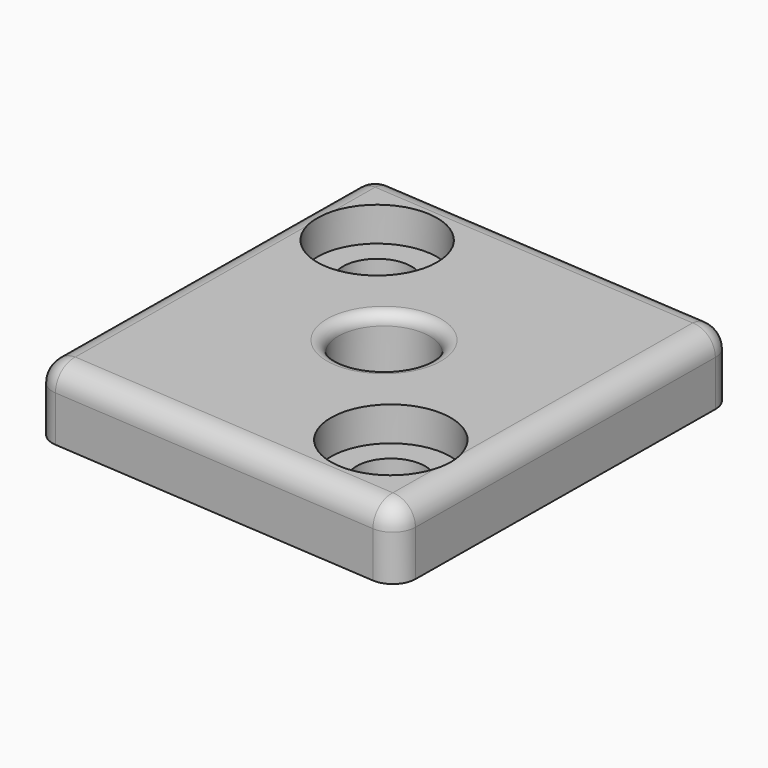
from build123d import *

# Parameters (mm, degrees)
F0_R         = 2.625
F0_R_2       = 2
F0_R_3       = 1.5
F1_DEPTH     = 3
F2_R         = 2.625
F2_R_2       = 1.5
F3_DEPTH     = 1.5
F4_T1_DEPTH  = 16.2344954865
F4_T3_DEPTH  = 14.8006020278
F4_T5_DEPTH  = 16.2344954865
F4_T7_DEPTH  = 14.8006020278
F4_T9_DEPTH  = 4.3472443006
F4_T11_DEPTH = 4.6626968477
F4_T16_DEPTH = 1
F4_T22_DEPTH = 1
F4_T28_DEPTH = 1
F4_T34_DEPTH = 1
F5_R         = 0.5


# Not quite as in the source:
# - a fillet or chamfer that OpenCascade refuses, or shapes differently, is made with other operations: its cross-section is extruded or revolved along the edge and cut away or added


with BuildPart() as f1:
    # F0 (on Top) → F1 (new body)
    with BuildSketch(Plane.XY):
        Polygon((8.4645454874, 8.5124193832), (-8.2962074114, 9.7252756798), (-8.4645454874, -8.5124193832), (8.2962074114, -9.7252756798), align=None)
        with Locations((4.8033426305, -5.6307453454)):
            Circle(F0_R, mode=Mode.SUBTRACT)
        Polygon((-2.3040371523, -3.3198032774), (-4.02705255, 0.3354530665), (-1.7230153977, 3.6552563439), (2.3040371523, 3.3198032774), (4.02705255, -0.3354530665), (1.7230153977, -3.6552563439), align=None, mode=Mode.SUBTRACT)
        with Locations((-4.8033426305, 5.6307453454)):
            Circle(F0_R, mode=Mode.SUBTRACT)
        Polygon((-1.7230153977, 3.6552563439), (-4.02705255, 0.3354530665), (-2.3040371523, -3.3198032774), (1.7230153977, -3.6552563439), (4.02705255, -0.3354530665), (2.3040371523, 3.3198032774), align=None)
        Circle(F0_R_2, mode=Mode.SUBTRACT)
        with Locations((-4.8033426305, 5.6307453454)):
            Circle(F0_R)
        with Locations((-4.8033426305, 5.6307453454)):
            Circle(F0_R_3, mode=Mode.SUBTRACT)
        with Locations((4.8033426305, -5.6307453454)):
            Circle(F0_R)
        with Locations((4.8033426305, -5.6307453454)):
            Circle(F0_R_3, mode=Mode.SUBTRACT)
    extrude(amount=F1_DEPTH)

    # F2 (on face) → F3 (cut)
    with BuildSketch(Plane.XY.offset(3)):
        with Locations((-4.8033426305, 5.6307453454)):
            Circle(F2_R)
        with Locations((-4.8033426305, 5.6307453454)):
            Circle(F2_R_2, mode=Mode.SUBTRACT)
        with Locations((4.8033426305, -5.6307453454)):
            Circle(F2_R)
        with Locations((4.8033426305, -5.6307453454)):
            Circle(F2_R_2, mode=Mode.SUBTRACT)
    extrude(amount=-F3_DEPTH, mode=Mode.SUBTRACT)

    # F4: fillet of radius 1 on 8 edges, made by hand

    # F4_s2 → F4_t1 (cut)
    with BuildSketch(Plane(origin=(0.0792216076, 8.582844455, 0), x_dir=(0, 0, 1), z_dir=(-0.0092298344, -0.9999574042, 0))):
        with BuildLine():
            ThreePointArc((2, 8.3856167117), (2.7071067812, 8.0927234929), (3, 7.3856167117))
            Line((3, 7.3856167117), (3, 8.3856167117))
            Line((3, 8.3856167117), (2, 8.3856167117))
        make_face()
    extrude(amount=F4_T1_DEPTH, mode=Mode.SUBTRACT)

    # F4_s4 → F4_t3 (cut)
    with BuildSketch(Plane(origin=(6.8712291985, -0.4972219118, 0), x_dir=(0, 0, 1), z_dir=(-0.9973920448, 0.0721741576, 0))):
        with BuildLine():
            ThreePointArc((3, 8.1011408148), (2.7071067812, 8.808247596), (2, 9.1011408148))
            Line((2, 9.1011408148), (3, 9.1011408148))
            Line((3, 9.1011408148), (3, 8.1011408148))
        make_face()
    extrude(amount=F4_T3_DEPTH, mode=Mode.SUBTRACT)

    # F4_s6 → F4_t5 (cut)
    with BuildSketch(Plane(origin=(-0.0792216076, -8.582844455, 0), x_dir=(0, 0, 1), z_dir=(0.0092298344, 0.9999574042, 0))):
        with BuildLine():
            ThreePointArc((2, 8.3856167117), (2.7071067812, 8.0927234929), (3, 7.3856167117))
            Line((3, 7.3856167117), (3, 8.3856167117))
            Line((3, 8.3856167117), (2, 8.3856167117))
        make_face()
    extrude(amount=F4_T5_DEPTH, mode=Mode.SUBTRACT)

    # F4_s8 → F4_t7 (cut)
    with BuildSketch(Plane(origin=(-6.8712291985, 0.4972219118, 0), x_dir=(0, 0, 1), z_dir=(0.9973920448, -0.0721741576, 0))):
        with BuildLine():
            ThreePointArc((2, 9.1011408148), (2.7071067812, 8.808247596), (3, 8.1011408148))
            Line((3, 8.1011408148), (3, 9.1011408148))
            Line((3, 9.1011408148), (2, 9.1011408148))
        make_face()
    extrude(amount=F4_T7_DEPTH, mode=Mode.SUBTRACT)

    # F4_s10 → F4_t9 (cut)
    with BuildSketch(Plane.XY.offset(-2.3472443006)):
        with BuildLine():
            ThreePointArc((8.4558796169, 7.573561656), (8.1912373991, 8.2605167863), (7.5280963703, 8.5801835352))
            Line((7.5280963703, 8.5801835352), (8.4645454874, 8.5124193832))
            Line((8.4645454874, 8.5124193832), (8.4558796169, 7.573561656))
        make_face()
        with BuildLine():
            ThreePointArc((-7.5280963703, -8.5801835352), (-8.1912373991, -8.2605167863), (-8.4558796169, -7.573561656))
            Line((-8.4558796169, -7.573561656), (-8.4645454874, -8.5124193832))
            Line((-8.4645454874, -8.5124193832), (-7.5280963703, -8.5801835352))
        make_face()
    extrude(amount=F4_T9_DEPTH, mode=Mode.SUBTRACT)

    # F4_s12 → F4_t11 (cut)
    with BuildSketch(Plane.XY.offset(-2.6626968477)):
        with BuildLine():
            ThreePointArc((7.23390635, -9.648404519), (7.9838058035, -9.3863276607), (8.3060379118, -8.6602423087))
            Line((8.3060379118, -8.6602423087), (8.2962074114, -9.7252756798))
            Line((8.2962074114, -9.7252756798), (7.23390635, -9.648404519))
        make_face()
        with BuildLine():
            ThreePointArc((-8.3060379118, 8.6602423087), (-7.9838058035, 9.3863276607), (-7.23390635, 9.648404519))
            Line((-7.23390635, 9.648404519), (-8.2962074114, 9.7252756798))
            Line((-8.2962074114, 9.7252756798), (-8.3060379118, 8.6602423087))
        make_face()
    extrude(amount=F4_T11_DEPTH, mode=Mode.SUBTRACT)


with BuildPart() as f4_tool14:
    # F4_s15 → F4_t16 (new body)
    with BuildSketch(Plane.XY.offset(2)):
        Polygon((-7.3060805076, 8.6510124742), (-7.23390635, 9.648404519), (-8.2962074114, 9.7252756798), (-8.3060379118, 8.6602423087), align=None)
    extrude(amount=F4_T16_DEPTH)

    # F4_s17 → F4_t18 (revolve, cut)
    with BuildSketch(Plane(origin=(-7.3060805076, 8.6510124742, 2), x_dir=(0.6777252959, -0.7353151864, 0), z_dir=(-0.7353151864, -0.6777252959, 0))):
        with BuildLine():
            ThreePointArc((0, -1), (1, 0), (0, 1))
            Line((0, 1), (0, -1))
        make_face()
    revolve(axis=Axis((-7.3060805076, 8.6510124742, 2), (0, 0, 1)), mode=Mode.SUBTRACT)


with BuildPart() as f1_1:
    add(f1.part)

    # F4_t13: cut F4_tool14
    add(f4_tool14.part, mode=Mode.SUBTRACT)


with BuildPart() as f4_tool20:
    # F4_s21 → F4_t22 (new body)
    with BuildSketch(Plane.XY.offset(2)):
        Polygon((-7.4559222127, -7.5827914904), (-7.5280963703, -8.5801835352), (-8.4645454874, -8.5124193832), (-8.4558796169, -7.573561656), align=None)
    extrude(amount=F4_T22_DEPTH)

    # F4_s23 → F4_t24 (revolve, cut)
    with BuildSketch(Plane(origin=(-7.4559222127, -7.5827914904, 2), x_dir=(0.7353151864, 0.6777252959, 0), z_dir=(0.6777252959, -0.7353151864, 0))):
        with BuildLine():
            ThreePointArc((0, -1), (1, 0), (0, 1))
            Line((0, 1), (0, -1))
        make_face()
    revolve(axis=Axis((-7.4559222127, -7.5827914904, 2), (0, 0, 1)), mode=Mode.SUBTRACT)


with BuildPart() as f1_2:
    add(f1_1.part)

    # F4_t19: cut F4_tool20
    add(f4_tool20.part, mode=Mode.SUBTRACT)


with BuildPart() as f4_tool26:
    # F4_s27 → F4_t28 (new body)
    with BuildSketch(Plane.XY.offset(2)):
        Polygon((7.4559222127, 7.5827914904), (7.5280963703, 8.5801835352), (8.4645454874, 8.5124193832), (8.4558796169, 7.573561656), align=None)
    extrude(amount=F4_T28_DEPTH)

    # F4_s29 → F4_t30 (revolve, cut)
    with BuildSketch(Plane(origin=(7.4559222127, 7.5827914904, 2), x_dir=(-0.7353151864, -0.6777252959, 0), z_dir=(-0.6777252959, 0.7353151864, 0))):
        with BuildLine():
            ThreePointArc((0, -1), (1, 0), (0, 1))
            Line((0, 1), (0, -1))
        make_face()
    revolve(axis=Axis((7.4559222127, 7.5827914904, 2), (0, 0, 1)), mode=Mode.SUBTRACT)


with BuildPart() as f1_3:
    add(f1_2.part)

    # F4_t25: cut F4_tool26
    add(f4_tool26.part, mode=Mode.SUBTRACT)


with BuildPart() as f4_tool32:
    # F4_s33 → F4_t34 (new body)
    with BuildSketch(Plane.XY.offset(2)):
        Polygon((7.3060805076, -8.6510124742), (7.23390635, -9.648404519), (8.2962074114, -9.7252756798), (8.3060379118, -8.6602423087), align=None)
    extrude(amount=F4_T34_DEPTH)

    # F4_s35 → F4_t36 (revolve, cut)
    with BuildSketch(Plane(origin=(7.3060805076, -8.6510124742, 2), x_dir=(-0.6777252959, 0.7353151864, 0), z_dir=(0.7353151864, 0.6777252959, 0))):
        with BuildLine():
            ThreePointArc((0, -1), (1, 0), (0, 1))
            Line((0, 1), (0, -1))
        make_face()
    revolve(axis=Axis((7.3060805076, -8.6510124742, 2), (0, 0, 1)), mode=Mode.SUBTRACT)


with BuildPart() as f1_4:
    add(f1_3.part)

    # F4_t31: cut F4_tool32
    add(f4_tool32.part, mode=Mode.SUBTRACT)

    # F5
    f5_edges = [f1_4.edges().sort_by_distance(p)[0] for p in [
        (-2, 0, 3),
    ]]
    fillet(f5_edges, radius=F5_R)


solid = f1_4.part
